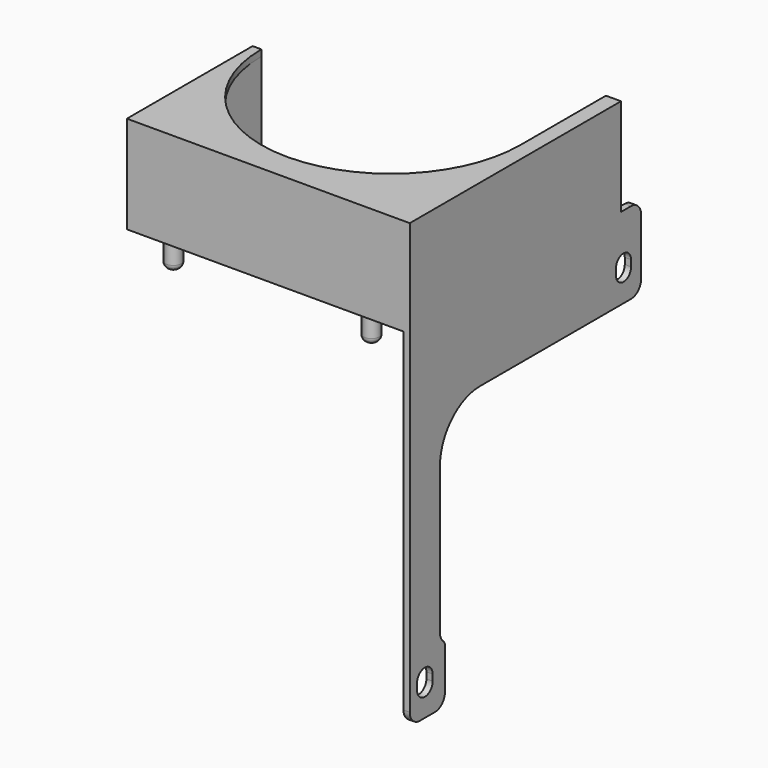
from build123d import *

# Parameters (mm, degrees)
F0_W         = 44
F0_H         = 42
F1_DEPTH     = 1
F3_DEPTH     = 13.5
F4_W         = 41.2
F4_H         = 40.1
F5_DEPTH     = 1
F7_DEPTH     = 25
F9_DEPTH     = 1
F11_DEPTH    = 25
F12_W        = 42
F12_H        = 15.5
F12_W_2      = 1
F12_H_2      = 9
F13_DEPTH    = 1
F14_DEPTH    = 25
F15_R        = 8
F16_T1_DEPTH = 1
F16_T3_DEPTH = 11
F16_T5_DEPTH = 11
F16_T7_DEPTH = 11
F16_T9_DEPTH = 11
F8_R         = 1.25
F17_DEPTH    = 5
F18_R        = 1


# Not quite as in the source:
# - a fillet or chamfer that OpenCascade refuses, or shapes differently, is made with other operations: its cross-section is extruded or revolved along the edge and cut away or added
# - a feature names something its author has since deleted; it is built from what else it names


with BuildPart() as f1:
    # F0 (on Top) → F1 (new body)
    with BuildSketch(Plane.XY):
        Rectangle(F0_W, F0_H)
    extrude(amount=F1_DEPTH)

    # F2 (on face) → F3 (join)
    with BuildSketch(Plane.XY.offset(1)):
        Polygon((-20.6, -19.1), (-20.6, 21), (-22, 21), (-22, -21), (22, -21), (22, 21), (20.6, 21), (20.6, -19.1), align=None)
    extrude(amount=F3_DEPTH)

    # F4 (on face) → F5 (join)
    with BuildSketch(Plane.XY.offset(14.5)):
        with Locations((0, 0.95)):
            Rectangle(F4_W, F4_H)
        Polygon((-22, 21), (-22, -21), (22, -21), (22, 21), (20.6, 21), (20.6, -19.1), (-20.6, -19.1), (-20.6, 21), align=None)
    extrude(amount=F5_DEPTH)

    # F6 (on face) → F7 (cut, symmetric)
    with BuildSketch(Plane.XY.offset(1)):
        with BuildLine():
            ThreePointArc((-20.6, 4.0000000362), (-1.81e-08, -16.6), (20.6, 4))
            ThreePointArc((20.6, 4), (18.2212690578, 13.6096490011), (11.6344316578, 21))
            Line((11.6344316578, 21), (-11.6344316578, 21))
            ThreePointArc((-11.6344316578, 21), (-18.2212690493, 13.6096490171), (-20.6, 4.0000000362))
        make_face()
        with BuildLine():
            Line((-20.6, 21), (-20.6, 4.0000000362))
            ThreePointArc((-20.6, 4.0000000362), (-18.2212690493, 13.6096490171), (-11.6344316578, 21))
            Line((-11.6344316578, 21), (-20.6, 21))
        make_face()
        with BuildLine():
            ThreePointArc((11.6344316578, 21), (18.2212690578, 13.6096490011), (20.6, 4))
            Line((20.6, 4), (20.6, 21))
            Line((20.6, 21), (11.6344316578, 21))
        make_face()
    extrude(amount=F7_DEPTH, both=True, mode=Mode.SUBTRACT)

    # F4 (on face) → F9 (join)
    with BuildSketch(Plane.XY.offset(14.5)):
        Polygon((-22, 21), (-22, -21), (22, -21), (22, 21), (20.6, 21), (20.6, -19.1), (-20.6, -19.1), (-20.6, 21), align=None)
    extrude(amount=F9_DEPTH)

    # F10 (on face) → F11 (cut)
    with BuildSketch(Plane.YZ.offset(-20.6)):
        Polygon((21, 0), (21, 15), (21, 15.5), (4, 15.5), (4, 14.5), (4, 1), (4, 0), align=None)
    extrude(amount=-F11_DEPTH, mode=Mode.SUBTRACT)

    # F12 (on face) → F13 (join)
    with BuildSketch(Plane.YZ.offset(22)):
        Polygon((21, 0), (-21, 0), (-21, -13), (-15, -13), (25, -13), (25, 0), align=None)
        with BuildLine():
            Line((23, -7.5), (23, -8.5))
            ThreePointArc((23, -8.5), (21.5, -10), (20, -8.5))
            Line((20, -8.5), (20, -7.5))
            ThreePointArc((20, -7.5), (21.5, -6), (23, -7.5))
        make_face(mode=Mode.SUBTRACT)
        Polygon((-15, -13), (-21, -13), (-21, -55), (-15, -55), (-15, -46), align=None)
        with BuildLine():
            Line((-16.45, -49.5), (-16.45, -50.5))
            ThreePointArc((-16.45, -50.5), (-18, -52.05), (-19.55, -50.5))
            Line((-19.55, -50.5), (-19.55, -49.5))
            ThreePointArc((-19.55, -49.5), (-18, -47.95), (-16.45, -49.5))
        make_face(mode=Mode.SUBTRACT)
        with Locations((0, 7.75)):
            Rectangle(F12_W, F12_H)
        with Locations((-14.5, -50.5)):
            Rectangle(F12_W_2, F12_H_2)
    extrude(amount=F13_DEPTH)

    # F12 (on face) → F14 (cut)
    with BuildSketch(Plane.YZ.offset(22)):
        with BuildLine():
            ThreePointArc((-19.55, -50.5), (-18, -52.05), (-16.45, -50.5))
            Line((-16.45, -50.5), (-16.8157280718, -50.5))
            ThreePointArc((-16.8157280718, -50.5), (-18, -51.05), (-19.1842719282, -50.5))
            Line((-19.1842719282, -50.5), (-19.55, -50.5))
        make_face()
        with BuildLine():
            Line((-16.8157280718, -50.5), (-16.45, -50.5))
            ThreePointArc((-16.45, -50.5), (-16.4708552854, -50.2465903676), (-16.5328599249, -50))
            ThreePointArc((-16.5328599249, -50), (-16.6509275769, -50.2632192327), (-16.8157280718, -50.5))
        make_face()
        with BuildLine():
            ThreePointArc((-16.5328599249, -50), (-16.4708552854, -50.2465903676), (-16.45, -50.5))
            Line((-16.45, -50.5), (-16.45, -49.5))
            ThreePointArc((-16.45, -49.5), (-16.4708552854, -49.7534096324), (-16.5328599249, -50))
        make_face()
        with BuildLine():
            ThreePointArc((-16.5328599249, -50), (-16.4708552854, -49.7534096324), (-16.45, -49.5))
            Line((-16.45, -49.5), (-16.8157280718, -49.5))
            ThreePointArc((-16.8157280718, -49.5), (-16.6509275769, -49.7367807673), (-16.5328599249, -50))
        make_face()
        with BuildLine():
            Line((-16.8157280718, -49.5), (-16.45, -49.5))
            ThreePointArc((-16.45, -49.5), (-18, -47.95), (-19.55, -49.5))
            Line((-19.55, -49.5), (-19.1842719282, -49.5))
            ThreePointArc((-19.1842719282, -49.5), (-18, -48.95), (-16.8157280718, -49.5))
        make_face()
        with BuildLine():
            Line((-19.1842719282, -49.5), (-16.8157280718, -49.5))
            ThreePointArc((-16.8157280718, -49.5), (-18, -48.95), (-19.1842719282, -49.5))
        make_face()
        with BuildLine():
            Line((-19.1842719282, -50.5), (-16.8157280718, -50.5))
            ThreePointArc((-16.8157280718, -50.5), (-16.6509275769, -50.2632192327), (-16.5328599249, -50))
            ThreePointArc((-16.5328599249, -50), (-16.6509275769, -49.7367807673), (-16.8157280718, -49.5))
            Line((-16.8157280718, -49.5), (-19.1842719282, -49.5))
            ThreePointArc((-19.1842719282, -49.5), (-19.3490724231, -49.7367807673), (-19.4671400751, -50))
            ThreePointArc((-19.4671400751, -50), (-19.3490724231, -50.2632192327), (-19.1842719282, -50.5))
        make_face()
        with BuildLine():
            ThreePointArc((-19.1842719282, -50.5), (-18, -51.05), (-16.8157280718, -50.5))
            Line((-16.8157280718, -50.5), (-19.1842719282, -50.5))
        make_face()
        with BuildLine():
            ThreePointArc((-19.4671400751, -50), (-19.5291447146, -50.2465903676), (-19.55, -50.5))
            Line((-19.55, -50.5), (-19.1842719282, -50.5))
            ThreePointArc((-19.1842719282, -50.5), (-19.3490724231, -50.2632192327), (-19.4671400751, -50))
        make_face()
        with BuildLine():
            Line((-19.55, -49.5), (-19.55, -50.5))
            ThreePointArc((-19.55, -50.5), (-19.5291447146, -50.2465903676), (-19.4671400751, -50))
            ThreePointArc((-19.4671400751, -50), (-19.5291447146, -49.7534096324), (-19.55, -49.5))
        make_face()
        with BuildLine():
            Line((-19.1842719282, -49.5), (-19.55, -49.5))
            ThreePointArc((-19.55, -49.5), (-19.5291447146, -49.7534096324), (-19.4671400751, -50))
            ThreePointArc((-19.4671400751, -50), (-19.3490724231, -49.7367807673), (-19.1842719282, -49.5))
        make_face()
        with BuildLine():
            ThreePointArc((20, -8.5), (21.5, -10), (23, -8.5))
            Line((23, -8.5), (22.6180339887, -8.5))
            ThreePointArc((22.6180339887, -8.5), (21.5, -9), (20.3819660113, -8.5))
            Line((20.3819660113, -8.5), (20, -8.5))
        make_face()
        with BuildLine():
            ThreePointArc((20.0857864376, -8), (20.0216021605, -8.2463470319), (20, -8.5))
            Line((20, -8.5), (20.3819660113, -8.5))
            ThreePointArc((20.3819660113, -8.5), (20.209430585, -8.2644805982), (20.0857864376, -8))
        make_face()
        with BuildLine():
            Line((20.3819660113, -7.5), (20, -7.5))
            ThreePointArc((20, -7.5), (20.0216021605, -7.7536529681), (20.0857864376, -8))
            ThreePointArc((20.0857864376, -8), (20.209430585, -7.7355194018), (20.3819660113, -7.5))
        make_face()
        with BuildLine():
            Line((22.6180339887, -7.5), (23, -7.5))
            ThreePointArc((23, -7.5), (21.5, -6), (20, -7.5))
            Line((20, -7.5), (20.3819660113, -7.5))
            ThreePointArc((20.3819660113, -7.5), (21.5, -7), (22.6180339887, -7.5))
        make_face()
        with BuildLine():
            Line((20.3819660113, -7.5), (22.6180339887, -7.5))
            ThreePointArc((22.6180339887, -7.5), (21.5, -7), (20.3819660113, -7.5))
        make_face()
        with BuildLine():
            Line((20.3819660113, -8.5), (22.6180339887, -8.5))
            ThreePointArc((22.6180339887, -8.5), (22.790569415, -8.2644805982), (22.9142135624, -8))
            ThreePointArc((22.9142135624, -8), (22.790569415, -7.7355194018), (22.6180339887, -7.5))
            Line((22.6180339887, -7.5), (20.3819660113, -7.5))
            ThreePointArc((20.3819660113, -7.5), (20.209430585, -7.7355194018), (20.0857864376, -8))
            ThreePointArc((20.0857864376, -8), (20.209430585, -8.2644805982), (20.3819660113, -8.5))
        make_face()
        with BuildLine():
            ThreePointArc((20.3819660113, -8.5), (21.5, -9), (22.6180339887, -8.5))
            Line((22.6180339887, -8.5), (20.3819660113, -8.5))
        make_face()
        with BuildLine():
            ThreePointArc((22.9142135624, -8), (22.9783978395, -8.2463470319), (23, -8.5))
            Line((23, -8.5), (23, -7.5))
            ThreePointArc((23, -7.5), (22.9783978395, -7.7536529681), (22.9142135624, -8))
        make_face()
        with BuildLine():
            ThreePointArc((22.9142135624, -8), (22.9783978395, -7.7536529681), (23, -7.5))
            Line((23, -7.5), (22.6180339887, -7.5))
            ThreePointArc((22.6180339887, -7.5), (22.790569415, -7.7355194018), (22.9142135624, -8))
        make_face()
        with BuildLine():
            Line((22.6180339887, -8.5), (23, -8.5))
            ThreePointArc((23, -8.5), (22.9783978395, -8.2463470319), (22.9142135624, -8))
            ThreePointArc((22.9142135624, -8), (22.790569415, -8.2644805982), (22.6180339887, -8.5))
        make_face()
        with BuildLine():
            Line((20, -7.5), (20, -8.5))
            ThreePointArc((20, -8.5), (20.0216021605, -8.2463470319), (20.0857864376, -8))
            ThreePointArc((20.0857864376, -8), (20.0216021605, -7.7536529681), (20, -7.5))
        make_face()
    extrude(amount=-F14_DEPTH, mode=Mode.SUBTRACT)

    # F15
    f15_edges = [f1.edges().sort_by_distance(p)[0] for p in [
        (22.5, -15, -13),
    ]]
    fillet(f15_edges, radius=F15_R)

    # F16: fillet of radius 2 on 5 edges, made by hand

    # F16_s2 → F16_t1 (join)
    with BuildSketch(Plane.YZ.offset(22)):
        with BuildLine():
            ThreePointArc((-15, -44.2679491924), (-14.7320508076, -45.2679491924), (-14, -46))
            Line((-14, -46), (-15, -46))
            Line((-15, -46), (-15, -44.2679491924))
        make_face()
    extrude(amount=F16_T1_DEPTH)

    # F16_s4 → F16_t3 (cut)
    with BuildSketch(Plane.YZ.offset(17)):
        with BuildLine():
            ThreePointArc((23, -13), (24.4142135624, -12.4142135624), (25, -11))
            Line((25, -11), (25, -13))
            Line((25, -13), (23, -13))
        make_face()
    extrude(amount=F16_T3_DEPTH, mode=Mode.SUBTRACT)

    # F16_s6 → F16_t5 (cut)
    with BuildSketch(Plane.YZ.offset(17)):
        with BuildLine():
            ThreePointArc((23, 0), (24.4142135624, -0.5857864376), (25, -2))
            Line((25, -2), (25, 0))
            Line((25, 0), (23, 0))
        make_face()
    extrude(amount=F16_T5_DEPTH, mode=Mode.SUBTRACT)

    # F16_s8 → F16_t7 (cut)
    with BuildSketch(Plane.YZ.offset(17)):
        with BuildLine():
            ThreePointArc((-14, -53), (-14.5857864376, -54.4142135624), (-16, -55))
            Line((-16, -55), (-14, -55))
            Line((-14, -55), (-14, -53))
        make_face()
    extrude(amount=F16_T7_DEPTH, mode=Mode.SUBTRACT)

    # F16_s10 → F16_t9 (cut)
    with BuildSketch(Plane.YZ.offset(17)):
        with BuildLine():
            ThreePointArc((-19, -55), (-20.4142135624, -54.4142135624), (-21, -53))
            Line((-21, -53), (-21, -55))
            Line((-21, -55), (-19, -55))
        make_face()
    extrude(amount=F16_T9_DEPTH, mode=Mode.SUBTRACT)

    # F8 (on face) → F17 (join)
    with BuildSketch(Plane(origin=(0, 0, 0), x_dir=(1, 0, 0), z_dir=(0, 0, -1))):
        with Locations((-17, 18)):
            Circle(F8_R)
        with Locations((14.5, 18)):
            Circle(F8_R)
    extrude(amount=F17_DEPTH)

    # F18
    f18_edges = [f1.edges().sort_by_distance(p)[0] for p in [
        (-18.25, -18, -5),
        (13.25, -18, -5),
        (22.5, -14, -46),
    ]]
    fillet(f18_edges, radius=F18_R)


solid = f1.part
